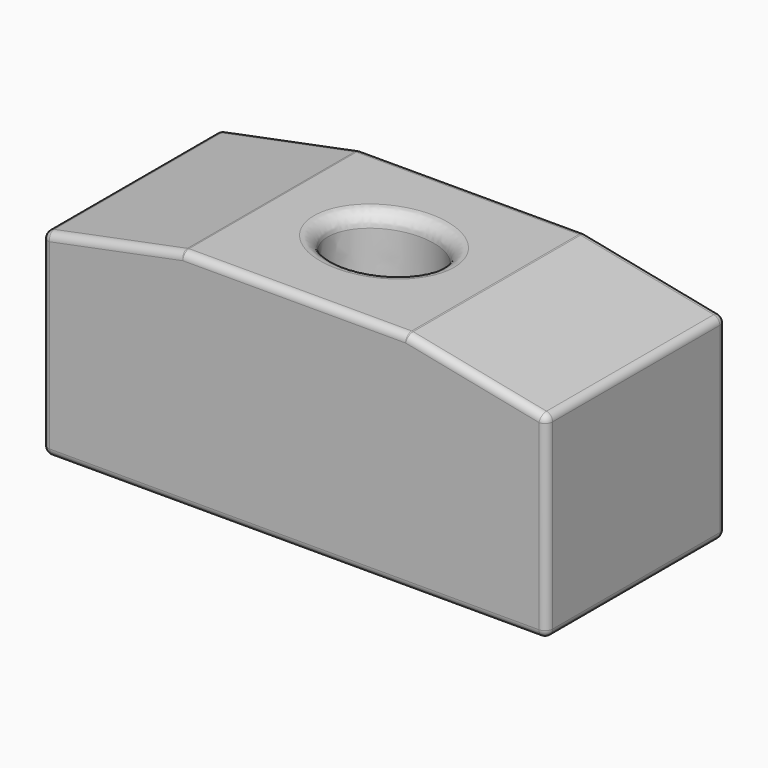
from build123d import *

# Parameters (mm, degrees)
F0_W     = 114.3
F0_H     = 50.8
F1_DEPTH = 50.8
F3_DEPTH = 50.801
F4_R     = 3.175
F6_DEPTH = 50.8010001
F7_R     = 1.7145


with BuildPart() as f1:
    # F0 (on Front) → F1 (new body)
    with BuildSketch(Plane.XZ):
        with Locations((57.15, 25.4)):
            Rectangle(F0_W, F0_H)
    extrude(amount=F1_DEPTH)

    # F2 (on face) → F3 (cut, through all)
    with BuildSketch(Plane.XY.offset(50.8)):
        with BuildLine():
            add(Edge.make_bspline(
                [(69.85, -25.4), (69.85, -7.8023637951), (50.8, -16.6011818976), (31.75, -25.4), (50.8, -34.1988181024), (69.85, -42.9976362049), (69.85, -25.4)],
                knots=[0, 0, 0, 2.0943951024, 2.0943951024, 4.1887902048, 4.1887902048, 6.2831853072, 6.2831853072, 6.2831853072], degree=2, weights=[1, 0.5, 1, 0.5, 1, 0.5, 1]))
        make_face()
    extrude(amount=-F3_DEPTH, mode=Mode.SUBTRACT)

    # F4
    f4_edges = [f1.edges().sort_by_distance(p)[0] for p in [
        (44.45, -25.4, 50.8),
        (69.85, -25.4, 25.4),
        (44.45, -25.4, 0),
    ]]
    fillet(f4_edges, radius=F4_R)

    # F5 (on face) → F6 (cut, through all)
    with BuildSketch(Plane.XZ.offset(50.8)):
        Polygon((0, 44.45), (31.75, 50.8), (82.55, 50.8), (114.3, 44.45), (114.3, 57.15), (0, 57.15), align=None)
    extrude(amount=-F6_DEPTH, mode=Mode.SUBTRACT)

    # F7
    f7_edges = [f1.edges().sort_by_distance(p)[0] for p in [
        (15.875, -50.8, 47.625),
        (31.75, -25.4, 50.8),
        (15.875, 0, 47.625),
        (0, -25.4, 44.45),
        (57.15, 0, 50.8),
        (57.15, -50.8, 50.8),
        (82.55, -25.4, 50.8),
        (41.275, -25.4, 50.8),
        (98.425, -50.8, 47.625),
        (114.3, -25.4, 44.45),
        (98.425, 0, 47.625),
        (114.3, -50.8, 22.225),
        (57.15, -50.8, 0),
        (0, -50.8, 22.225),
        (114.3, 0, 22.225),
        (114.3, -25.4, 0),
        (57.15, 0, 0),
        (0, 0, 22.225),
        (41.275, -25.4, 0),
        (0, -25.4, 0),
    ]]
    fillet(f7_edges, radius=F7_R)


solid = f1.part
